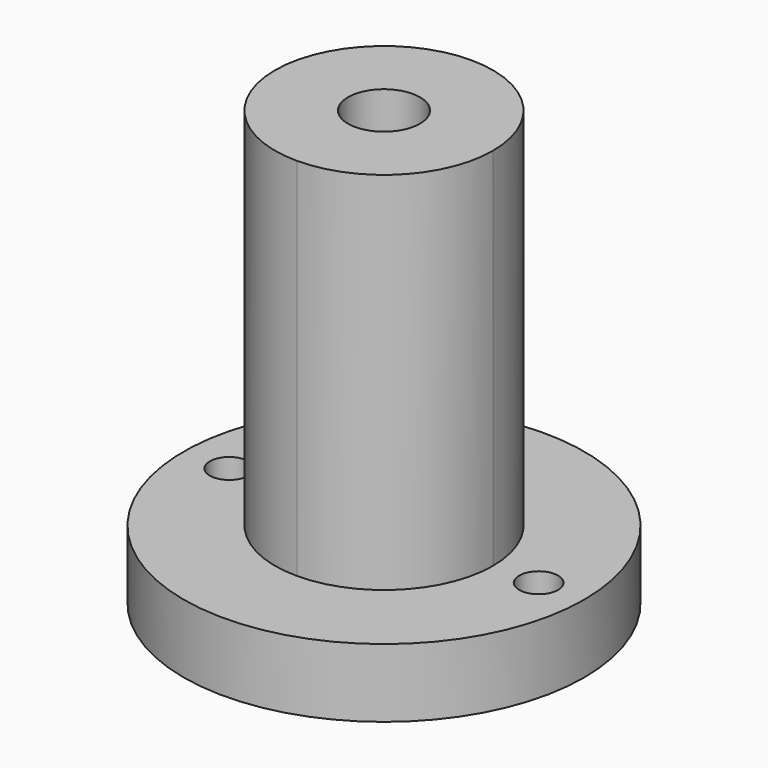
from build123d import *

# Parameters (mm, degrees)
F0_W        = 15.1496281502
F0_H        = 15.1496281502
F0_R        = 2.5
F1_DEPTH    = 25.4
F2_R        = 1.7272
F3_REACH    = 20.0358874801
F4_R        = 13.9248140751
F4_R_2      = 1.35255
F4_R_3      = 2.5
F5_DEPTH    = 4.7625
F6_T1_DEPTH = 44.3370335


# Not quite as in the source:
# - a fillet or chamfer that OpenCascade refuses, or shapes differently, is made with other operations: its cross-section is extruded or revolved along the edge and cut away or added


with BuildPart() as f1:
    # F0 (on Top) → F1 (new body)
    with BuildSketch(Plane.XY):
        Rectangle(F0_W, F0_H)
        Circle(F0_R, mode=Mode.SUBTRACT)
    extrude(amount=F1_DEPTH)

    f3_end = f1.faces().sort_by_distance((-2.5, 0, 12.7))[0]
    # F2 (on face) → F3 (cut, up to a face of the model that its end follows)
    with BuildSketch(Plane(origin=(0, 7.5748140751, 0), x_dir=(-1, 0, 0), z_dir=(0, 1, 0))):
        with Locations((0, 12.7)):
            Circle(F2_R)
    f3_long = extrude(amount=-F3_REACH, mode=Mode.PRIVATE)
    add(split(f3_long, bisect_by=f3_end, keep=Keep.ALL, mode=Mode.PRIVATE).solids().sort_by_distance((0, 7.5748140751, 12.7))[0], mode=Mode.SUBTRACT)

    # F4 (on face) → F5 (join)
    with BuildSketch(Plane(origin=(0, 0, 0), x_dir=(1, 0, 0), z_dir=(0, 0, -1))):
        Circle(F4_R)
        with Locations((-10.7498140751, 0)):
            Circle(F4_R_2, mode=Mode.SUBTRACT)
        Circle(F4_R_3, mode=Mode.SUBTRACT)
        with Locations((10.7498140751, 0)):
            Circle(F4_R_2, mode=Mode.SUBTRACT)
    extrude(amount=F5_DEPTH)

    # F6: fillet of radius 7.5748134 on 4 edges, made by hand

    # F6_s2 → F6_t1 (cut)
    with BuildSketch(Plane.XY):
        with BuildLine():
            ThreePointArc((-6.751e-07, 7.5748140751), (-5.3562025965, 5.3562025965), (-7.5748140751, 6.751e-07))
            Line((-7.5748140751, 6.751e-07), (-7.5748140751, 7.5748140751))
            Line((-7.5748140751, 7.5748140751), (-6.751e-07, 7.5748140751))
        make_face()
        with BuildLine():
            ThreePointArc((6.751e-07, 7.5748140751), (5.3562025965, 5.3562025965), (7.5748140751, 6.751e-07))
            Line((7.5748140751, 6.751e-07), (7.5748140751, 7.5748140751))
            Line((7.5748140751, 7.5748140751), (6.751e-07, 7.5748140751))
        make_face()
        with BuildLine():
            ThreePointArc((-6.751e-07, -7.5748140751), (-5.3562025965, -5.3562025965), (-7.5748140751, -6.751e-07))
            Line((-7.5748140751, -6.751e-07), (-7.5748140751, -7.5748140751))
            Line((-7.5748140751, -7.5748140751), (-6.751e-07, -7.5748140751))
        make_face()
        with BuildLine():
            ThreePointArc((6.751e-07, -7.5748140751), (5.3562025965, -5.3562025965), (7.5748140751, -6.751e-07))
            Line((7.5748140751, -6.751e-07), (7.5748140751, -7.5748140751))
            Line((7.5748140751, -7.5748140751), (6.751e-07, -7.5748140751))
        make_face()
    extrude(amount=F6_T1_DEPTH, mode=Mode.SUBTRACT)


solid = f1.part
